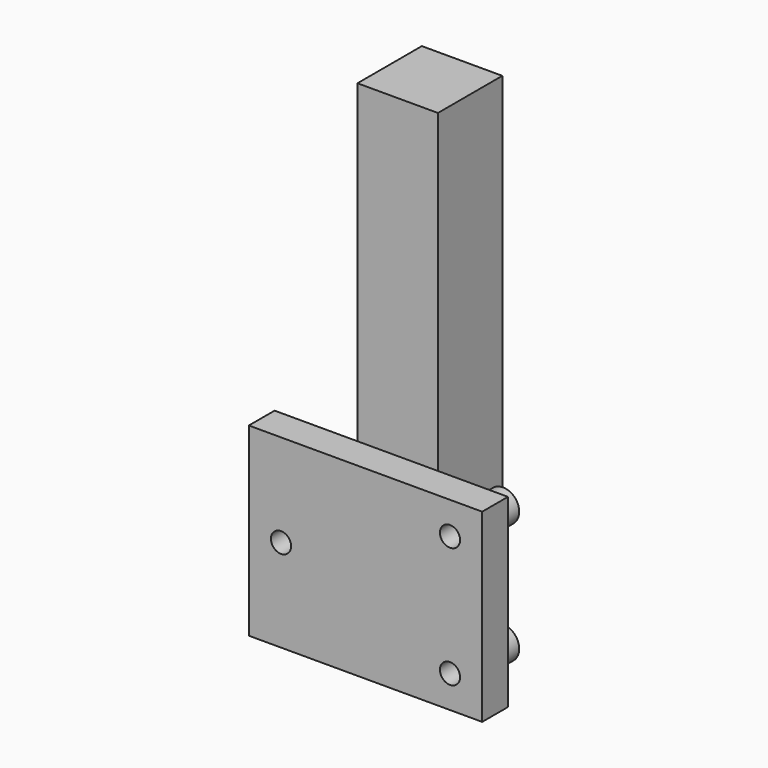
from build123d import *

# Parameters (mm, degrees)
F1_W     = 20
F1_H     = 20
F2_DEPTH = 100
F3_W     = 58
F3_H     = 46
F3_R     = 2.5
F4_DEPTH = 8
F5_R     = 8
F5_R_2   = 2.5
F5_R_3   = 7.5801298939
F6_DEPTH = 2
F7_SIZE  = 1.99999
F8_R     = 4
F8_R_2   = 2.5
F9_DEPTH = 6.5


# Not quite as in the source:
# - a fillet or chamfer is up to 0.001 mm smaller than in the source, because OpenCascade refuses the exact size


with BuildPart() as f2:
    # F1 (on Top) → F2 (new body)
    with BuildSketch(Plane.XY):
        Rectangle(F1_W, F1_H)
    extrude(amount=F2_DEPTH)


with BuildPart() as f4:
    # F3 (on offset) → F4 (new body)
    with BuildSketch(Plane.XZ.offset(12)):
        Rectangle(F3_W, F3_H)
        with Locations((21, -15)):
            Circle(F3_R, mode=Mode.SUBTRACT)
        with Locations((-21, 0)):
            Circle(F3_R, mode=Mode.SUBTRACT)
        with Locations((21, 15)):
            Circle(F3_R, mode=Mode.SUBTRACT)
    extrude(amount=F4_DEPTH)

    # F5 (on face) → F6 (join)
    with BuildSketch(Plane(origin=(0, -12, 0), x_dir=(-1, 0, 0), z_dir=(0, 1, 0))):
        with Locations((-21, 15)):
            Circle(F5_R)
        with Locations((-21, 15)):
            Circle(F5_R_2, mode=Mode.SUBTRACT)
        with Locations((-21, -15)):
            Circle(F5_R)
        with Locations((-21, -15)):
            Circle(F5_R_2, mode=Mode.SUBTRACT)
        with Locations((21, 0)):
            Circle(F5_R_3)
        with Locations((21, 0)):
            Circle(F5_R_2, mode=Mode.SUBTRACT)
    extrude(amount=F6_DEPTH)

    # F7 (size 2 in the source; OpenCascade refuses exactly that, so slightly less here)
    f7_edges = [f4.edges().sort_by_distance(p)[0] for p in [
        (29, -10, 15),
        (-13.41987, -10, 0),
        (29, -10, -15),
    ]]
    chamfer(f7_edges, length=F7_SIZE)


with BuildPart() as f9:
    # F8 (on face) → F9 (new body)
    with BuildSketch(Plane(origin=(0, -10, 0), x_dir=(-1, 0, 0), z_dir=(0, 1, 0))):
        with Locations((-21, 15)):
            Circle(F8_R)
        with Locations((-21, 15)):
            Circle(F8_R_2, mode=Mode.SUBTRACT)
    extrude(amount=F9_DEPTH)


with BuildPart() as f9b:
    # F8 (on face) → F9, piece 2 (new body)
    with BuildSketch(Plane(origin=(0, -10, 0), x_dir=(-1, 0, 0), z_dir=(0, 1, 0))):
        with Locations((21, 0)):
            Circle(F8_R)
        with Locations((21, 0)):
            Circle(F8_R_2, mode=Mode.SUBTRACT)
    extrude(amount=F9_DEPTH)


with BuildPart() as f9c:
    # F8 (on face) → F9, piece 3 (new body)
    with BuildSketch(Plane(origin=(0, -10, 0), x_dir=(-1, 0, 0), z_dir=(0, 1, 0))):
        with Locations((-21, -15)):
            Circle(F8_R)
        with Locations((-21, -15)):
            Circle(F8_R_2, mode=Mode.SUBTRACT)
    extrude(amount=F9_DEPTH)


solid = Compound([f2.part, f4.part, f9.part, f9b.part, f9c.part])
